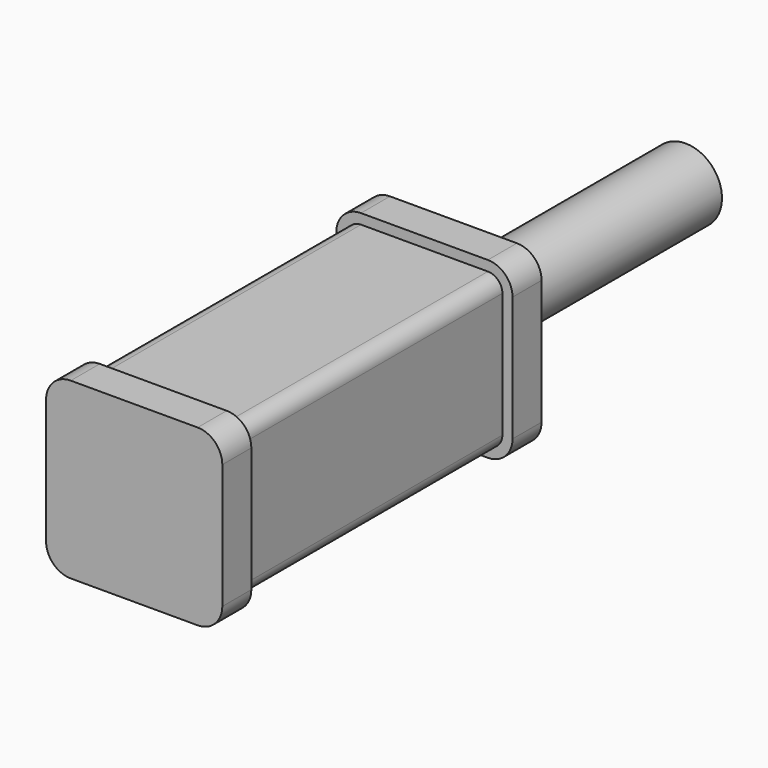
from build123d import *

# Parameters (mm, degrees)
F1_DEPTH = 250
F4_DEPTH = 25
F5_R     = 25.0490469986
F6_DEPTH = 200


with BuildPart() as f1:
    # F0 (on Front) → F1 (new body)
    with BuildSketch(Plane.XZ):
        with BuildLine():
            ThreePointArc((53.7174828351, 43.0048087239), (50.7885506469, 50.0758765358), (43.7174828351, 53.0048087239))
            Line((43.7174828351, 53.0048087239), (-43.7174828351, 53.0048087239))
            ThreePointArc((-43.7174828351, 53.0048087239), (-50.7885506469, 50.0758765358), (-53.7174828351, 43.0048087239))
            Line((-53.7174828351, 43.0048087239), (-53.7174828351, -43.0048087239))
            ThreePointArc((-53.7174828351, -43.0048087239), (-50.7885506469, -50.0758765358), (-43.7174828351, -53.0048087239))
            Line((-43.7174828351, -53.0048087239), (43.7174828351, -53.0048087239))
            ThreePointArc((43.7174828351, -53.0048087239), (50.7885506469, -50.0758765358), (53.7174828351, -43.0048087239))
            Line((53.7174828351, -43.0048087239), (53.7174828351, 43.0048087239))
        make_face()
    extrude(amount=F1_DEPTH)

    # F2 (on face) + F3 (on face) → F4 (join)
    with BuildSketch(Plane.XZ.offset(250)):
        with BuildLine():
            Line((-60.7174821198, 43.0048087239), (-60.7174821198, -43.0048087239))
            ThreePointArc((-60.7174821198, -43.0048087239), (-55.7382976095, -55.0256234983), (-43.7174828351, -60.0048080087))
            Line((-43.7174828351, -60.0048080087), (43.7174828351, -60.0048080087))
            ThreePointArc((43.7174828351, -60.0048080087), (55.7382976095, -55.0256234983), (60.7174821198, -43.0048087239))
            Line((60.7174821198, -43.0048087239), (60.7174821198, 43.0048087239))
            ThreePointArc((60.7174821198, 43.0048087239), (55.7382976095, 55.0256234983), (43.7174828351, 60.0048080087))
            Line((43.7174828351, 60.0048080087), (-43.7174828351, 60.0048080087))
            ThreePointArc((-43.7174828351, 60.0048080087), (-55.7382976095, 55.0256234983), (-60.7174821198, 43.0048087239))
        make_face()
    with BuildSketch(Plane(origin=(0, 0, 0), x_dir=(-1, 0, 0), z_dir=(0, 1, 0))):
        with BuildLine():
            Line((-60.7174821198, 43.0048087239), (-60.7174821198, -43.0048087239))
            ThreePointArc((-60.7174821198, -43.0048087239), (-55.7382976095, -55.0256234983), (-43.7174828351, -60.0048080087))
            Line((-43.7174828351, -60.0048080087), (43.7174828351, -60.0048080087))
            ThreePointArc((43.7174828351, -60.0048080087), (55.7382976095, -55.0256234983), (60.7174821198, -43.0048087239))
            Line((60.7174821198, -43.0048087239), (60.7174821198, 43.0048087239))
            ThreePointArc((60.7174821198, 43.0048087239), (55.7382976095, 55.0256234983), (43.7174828351, 60.0048080087))
            Line((43.7174828351, 60.0048080087), (-43.7174828351, 60.0048080087))
            ThreePointArc((-43.7174828351, 60.0048080087), (-55.7382976095, 55.0256234983), (-60.7174821198, 43.0048087239))
        make_face()
    extrude(amount=F4_DEPTH, dir=(0, -1, 0))

    # F5 (on face) → F6 (join)
    with BuildSketch(Plane(origin=(0, 0, 0), x_dir=(-1, 0, 0), z_dir=(0, 1, 0))):
        Circle(F5_R)
    extrude(amount=F6_DEPTH)


solid = f1.part
